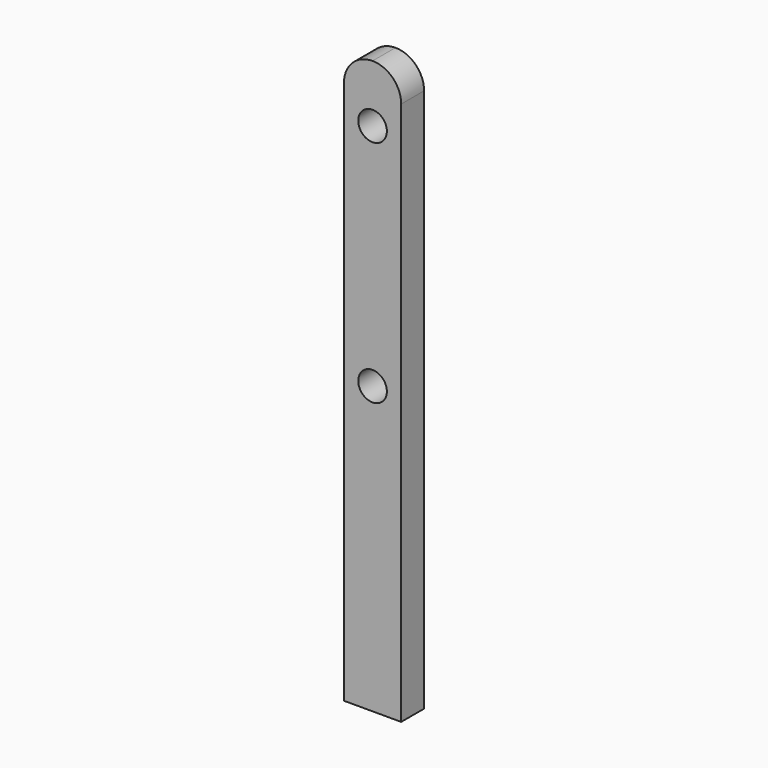
from build123d import *

# Parameters (mm, degrees)
F0_W     = 10
F0_H     = 100
F0_R     = 2.5
F1_DEPTH = 5
F2_R     = 4.99999


# Not quite as in the source:
# - a fillet or chamfer is up to 0.001 mm smaller than in the source, because OpenCascade refuses the exact size


with BuildPart() as f1:
    # F0 (on Front) → F1 (new body)
    with BuildSketch(Plane.XZ):
        with Locations((-43.9073760062, 47.7142522777)):
            Rectangle(F0_W, F0_H)
        with Locations((-43.9073760062, 47.7142522777)):
            Circle(F0_R, mode=Mode.SUBTRACT)
        with Locations((-43.9073760062, 87.7142522777)):
            Circle(F0_R, mode=Mode.SUBTRACT)
    extrude(amount=F1_DEPTH)

    # F2 (radius 5 in the source; OpenCascade refuses exactly that, so slightly less here)
    f2_edges = [f1.edges().sort_by_distance(p)[0] for p in [
        (-48.907376, -2.5, 97.714252),
        (-38.907376, -2.5, 97.714252),
    ]]
    fillet(f2_edges, radius=F2_R)


solid = f1.part
